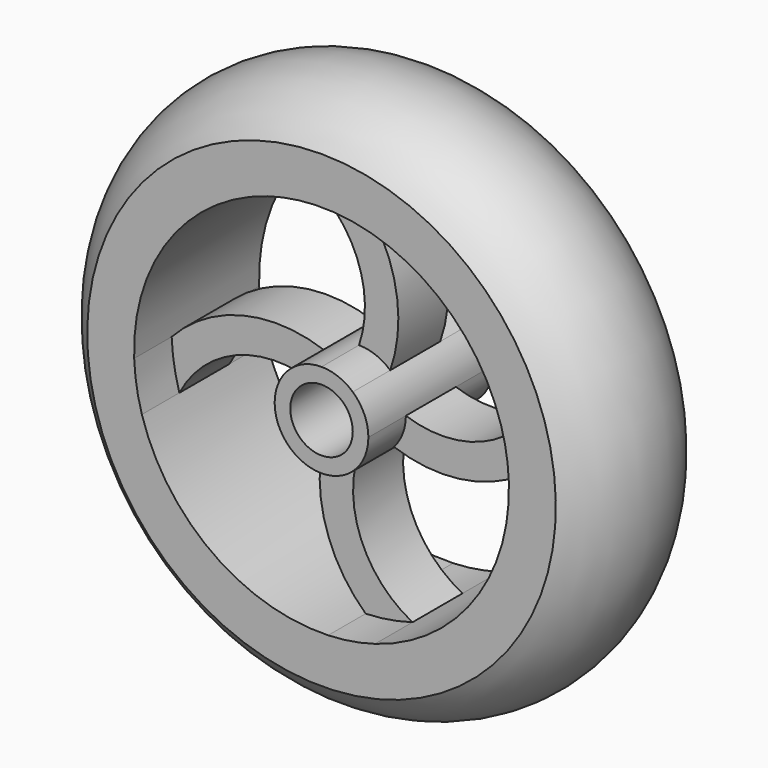
from build123d import *
from build123d import SkipClean  # not in build123d's __all__

# Parameters (mm, degrees)
F0_R     = 75
F0_R_2   = 10
F1_DEPTH = 50
F6_DEPTH = 15


# Not quite as in the source:
# - a pattern or mirror of a feature is missing from the dataset's text; its kind, count and spacing are read off the source's solid


with BuildPart() as f1:
    # F0 (on Front) → F1 (new body)
    with BuildSketch(Plane.XZ):
        Circle(F0_R)
        with BuildLine():
            ThreePointArc((-57.5027136201, -17.1300299569), (-39.4445240133, -0.6421875508), (-15, 0))
            ThreePointArc((-15, 0), (-13.6930639376, -6.123724357), (-10, -11.1803398875))
            ThreePointArc((-10, -11.1803398875), (-11.2445250944, -37.3888406037), (2.1300299569, -59.9621795166))
            ThreePointArc((2.1300299569, -59.9621795166), (-35.0025968036, -48.7321066342), (-57.5027136201, -17.1300299569))
        make_face(mode=Mode.SUBTRACT)
        with BuildLine():
            ThreePointArc((17.1300299569, -57.5027136201), (0.6421875508, -39.4445240133), (0, -15))
            ThreePointArc((0, -15), (6.123724357, -13.6930639376), (11.1803398875, -10))
            ThreePointArc((11.1803398875, -10), (37.3888406037, -11.2445250944), (59.9621795166, 2.1300299569))
            ThreePointArc((59.9621795166, 2.1300299569), (48.7321066342, -35.0025968036), (17.1300299569, -57.5027136201))
        make_face(mode=Mode.SUBTRACT)
        with BuildLine():
            ThreePointArc((-59.9621795166, -2.1300299569), (-48.7321066342, 35.0025968036), (-17.1300299569, 57.5027136201))
            ThreePointArc((-17.1300299569, 57.5027136201), (-0.6421875508, 39.4445240133), (0, 15))
            ThreePointArc((0, 15), (-6.123724357, 13.6930639376), (-11.1803398875, 10))
            ThreePointArc((-11.1803398875, 10), (-37.3888406037, 11.2445250944), (-59.9621795166, -2.1300299569))
        make_face(mode=Mode.SUBTRACT)
        Circle(F0_R_2, mode=Mode.SUBTRACT)
        with BuildLine():
            ThreePointArc((15, 0), (13.6930639376, 6.123724357), (10, 11.1803398875))
            ThreePointArc((10, 11.1803398875), (11.2445250944, 37.3888406037), (-2.1300299569, 59.9621795166))
            ThreePointArc((-2.1300299569, 59.9621795166), (35.0025968036, 48.7321066342), (57.5027136201, 17.1300299569))
            ThreePointArc((57.5027136201, 17.1300299569), (39.4445240133, 0.6421875508), (15, 0))
        make_face(mode=Mode.SUBTRACT)
    extrude(amount=F1_DEPTH)

    # F2 (on Right) → F3 (revolve)
    with BuildSketch(Plane.YZ):
        with BuildLine():
            Line((-50, 75), (0, 75))
            ThreePointArc((0, 75), (-25, 88.4168760482), (-50, 75))
        make_face()
    revolve(axis=Axis((0, -25, 0), (0, -1, 0)))

    # F5 (on face) → F6 (cut)
    with BuildSketch(Plane.XZ.offset(50)):
        with BuildLine():
            ThreePointArc((-17.1300299569, 57.5027136201), (-0.6421875508, 39.4445240133), (0, 15))
            ThreePointArc((0, 15), (5.3523313466, 14.0125853844), (10, 11.1803398875))
            ThreePointArc((10, 11.1803398875), (11.2445250944, 37.3888406037), (-2.1300299569, 59.9621795166))
            ThreePointArc((-2.1300299569, 59.9621795166), (-9.7082295036, 59.2093766215), (-17.1300299569, 57.5027136201))
        make_face()
        with BuildLine():
            ThreePointArc((57.5027136201, 17.1300299569), (39.4445240133, 0.6421875508), (15, 0))
            ThreePointArc((15, 0), (14.0125853844, -5.3523313466), (11.1803398875, -10))
            ThreePointArc((11.1803398875, -10), (37.3888406037, -11.2445250944), (59.9621795166, 2.1300299569))
            ThreePointArc((59.9621795166, 2.1300299569), (59.2093766215, 9.7082295036), (57.5027136201, 17.1300299569))
        make_face()
        with BuildLine():
            ThreePointArc((17.1300299569, -57.5027136201), (0.6421875508, -39.4445240133), (0, -15))
            ThreePointArc((0, -15), (-5.3523313466, -14.0125853844), (-10, -11.1803398875))
            ThreePointArc((-10, -11.1803398875), (-11.2445250944, -37.3888406037), (2.1300299569, -59.9621795166))
            ThreePointArc((2.1300299569, -59.9621795166), (9.7082295036, -59.2093766215), (17.1300299569, -57.5027136201))
        make_face()
        with BuildLine():
            ThreePointArc((-57.5027136201, -17.1300299569), (-39.4445240133, -0.6421875508), (-15, 0))
            ThreePointArc((-15, 0), (-14.0125853844, 5.3523313466), (-11.1803398875, 10))
            ThreePointArc((-11.1803398875, 10), (-37.3888406037, 11.2445250944), (-59.9621795166, -2.1300299569))
            ThreePointArc((-59.9621795166, -2.1300299569), (-59.2093766215, -9.7082295036), (-57.5027136201, -17.1300299569))
        make_face()
    with SkipClean():  # cleaning this boolean's faces spoils the solid; the shape is the same uncleaned
        f6 = extrude(amount=-F6_DEPTH, mode=Mode.SUBTRACT)

    # F6_copies: F6 across plane
    with SkipClean():  # cleaning this boolean's faces spoils the solid; the shape is the same uncleaned
        add(f6.mirror(Plane.ZX.offset(-25)), clean=False, mode=Mode.SUBTRACT)


solid = f1.part
